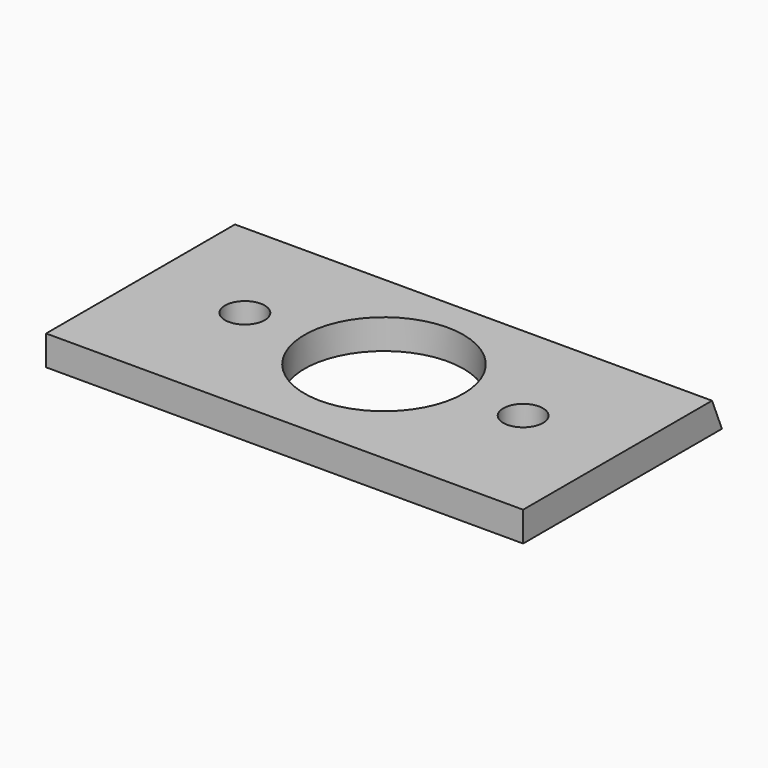
from build123d import *

# Parameters (mm, degrees)
F0_W     = 304.8
F0_H     = 158.75
F0_R     = 12.7
F0_R_2   = 50.8
F1_DEPTH = 19.05
F2_SIZE2 = 7.890758
F2_SIZE  = 19.04999


# Not quite as in the source:
# - a fillet or chamfer is up to 0.001 mm smaller than in the source, because OpenCascade refuses the exact size


with BuildPart() as f1:
    # F0 (on Top) → F1 (new body)
    with BuildSketch(Plane.XY):
        Rectangle(F0_W, F0_H)
        with Locations((-88.9, 0)):
            Circle(F0_R, mode=Mode.SUBTRACT)
        Circle(F0_R_2, mode=Mode.SUBTRACT)
        with BuildLine():
            ThreePointArc((88.9, -12.7), (79.9197438789, 8.9802561211), (101.6, 0))
            ThreePointArc((101.6, 0), (97.8802561211, -8.9802561211), (88.9, -12.7))
        make_face(mode=Mode.SUBTRACT)
    extrude(amount=F1_DEPTH)

    # F2 (size 19.05 and 7.8907683632 in the source; OpenCascade refuses exactly that, so slightly less here)
    f2_edges = [f1.edges().sort_by_distance(p)[0] for p in [
        (0, 79.375, 19.05),
    ]]
    f2_side = f1.faces().sort_by_distance((0, 79.375, 9.525))[0]
    chamfer(f2_edges, length=F2_SIZE, length2=F2_SIZE2, reference=f2_side)


solid = f1.part
